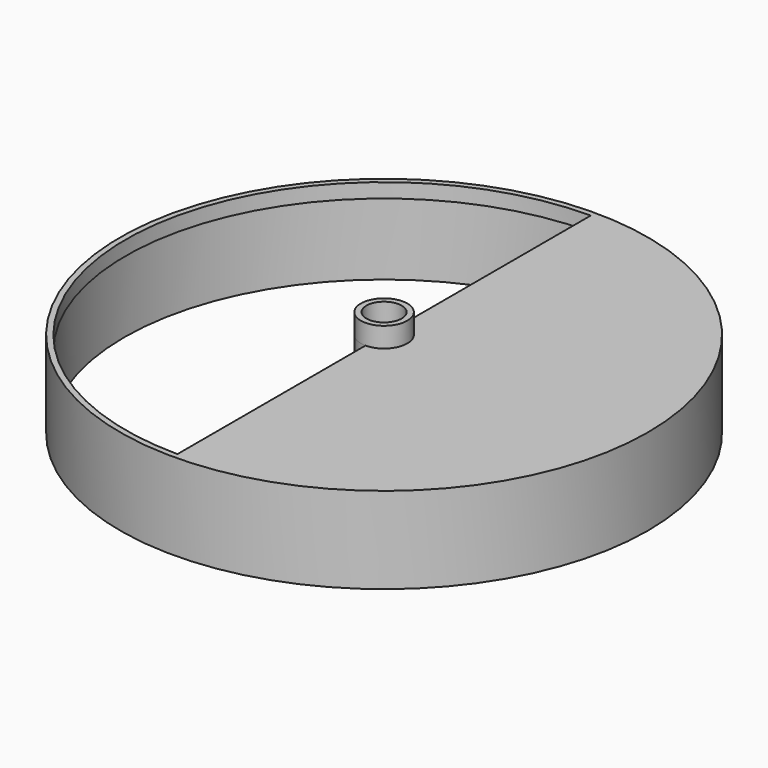
from build123d import *

# Parameters (mm, degrees)
F0_R          = 46.5
F1_DEPTH      = 15.24
F2_R          = 45.75
F3_DEPTH      = 12.7
F4_R          = 4.1
F5_DEPTH      = 3.53
F5_DEPTH_BACK = 1
F7_R          = 3.1
F8_DEPTH      = 18.771
F9_DEPTH      = 15.241


# Not quite as in the source:
# - after a boolean that leaves OpenCascade's solid faulty, fix() repairs it


with BuildPart() as f1:
    # F0 (on Top) → F1 (new body)
    with BuildSketch(Plane.XY):
        Circle(F0_R)
    extrude(amount=F1_DEPTH)

    # F2 (on Top) → F3 (cut)
    with BuildSketch(Plane.XY):
        Circle(F2_R)
    extrude(amount=F3_DEPTH, mode=Mode.SUBTRACT)

    # F4 (on face) → F5 (join, two sides)
    with BuildSketch(Plane.XY.offset(15.24)) as f5_sk:
        Circle(F4_R)
    extrude(amount=F5_DEPTH)
    extrude(f5_sk.sketch, amount=-F5_DEPTH_BACK)

    # F7 (on face) → F8 (cut, through all)
    with BuildSketch(Plane.XY.offset(18.77)):
        Circle(F7_R)
    extrude(amount=-F8_DEPTH, mode=Mode.SUBTRACT)

    # F6 (on face) → F9 (cut, through all)
    with BuildSketch(Plane.XY.offset(15.24)):
        with BuildLine():
            Line((0, 4.1), (0, 45.5))
            ThreePointArc((0, 45.5), (-45.5, 0), (0, -45.5))
            Line((0, -45.5), (0, -4.1))
            ThreePointArc((0, -4.1), (-4.1, 0), (0, 4.1))
        make_face()
    extrude(amount=-F9_DEPTH, mode=Mode.SUBTRACT)

    add(f1.part.fix(), mode=Mode.REPLACE)


solid = f1.part
